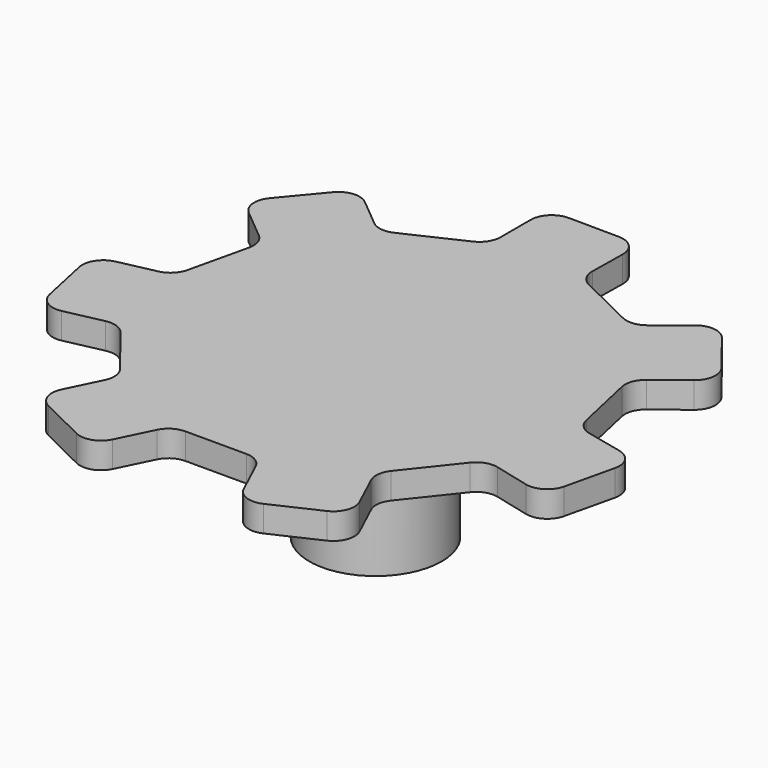
from build123d import *

# Parameters (mm, degrees)
F1_DEPTH  = 2.54
F2_SCALE  = 1.12
F3_R      = 1.27
F4_R      = 4.0005
F4_R_2    = 2.1462999284
F5_DEPTH  = 7.0104
F6_R      = 2.2083863112
F7_DEPTH  = 7.0104
F8_DEPTH  = 1.27
F9_R      = 5.1360331122
F10_DEPTH = 1.27


with BuildPart() as f1:
    # F0 (on Top) → F1 (new body)
    with BuildSketch(Plane.XY):
        Polygon((2.6097216178, 14.5627437159), (-2.4016266689, 14.6046923473), (-2.4016266689, 10.7069099322), (-6.7973635159, 8.6464090273), (-9.7507489845, 11.1018400639), (-12.9371215583, 7.269280193), (-9.9187448393, 4.759815731), (-10.987800546, 0.1461525389), (-14.7898914292, -0.6685812259), (-13.7329729143, -5.6008676039), (-9.9187448393, -4.7835330123), (-6.9650523365, -8.5103949532), (-8.662414737, -11.9730141014), (-4.136644538, -14.1915290003), (-2.4166579341, -10.6827564792), (2.3025460541, -10.6827564792), (3.9659612812, -14.2644541338), (8.5153820935, -12.1516080526), (6.8819414162, -8.6344521752), (9.8897544667, -4.8440932296), (13.6239528656, -5.7776425965), (14.7675592452, -0.8934023208), (10.9942825511, -0.0382388607), (9.9505092949, 4.6697063372), (13.008704409, 7.0334360935), (9.9016642198, 10.9836040065), (6.8838195875, 8.5752755404), (2.5481330231, 10.6975259259), align=None)
    extrude(amount=F1_DEPTH)


with BuildPart() as f1_1:
    # F2: moved
    add(f1.part.scale(F2_SCALE))

    # F3
    f3_edges = [f1_1.edges().sort_by_distance(p)[0] for p in [
        (-16.564678, -0.748811, 1.4224),
        (-12.306337, 0.163691, 1.4224),
        (-14.489576, 8.141594, 1.4224),
        (-10.920839, 12.434061, 1.4224),
        (-7.613047, 9.683978, 1.4224),
        (-2.689822, 11.991739, 1.4224),
        (-2.689822, 16.357255, 1.4224),
        (2.922888, 16.310273, 1.4224),
        (2.853909, 11.981229, 1.4224),
        (7.709878, 9.604309, 1.4224),
        (11.089864, 12.301636, 1.4224),
        (14.569749, 7.877448, 1.4224),
        (11.14457, 5.230071, 1.4224),
        (12.313596, -0.042828, 1.4224),
        (16.539666, -1.000611, 1.4224),
        (15.258827, -6.47096, 1.4224),
        (11.076525, -5.425384, 1.4224),
        (7.707774, -9.670586, 1.4224),
        (9.537228, -13.609801, 1.4224),
        (4.441877, -15.976189, 1.4224),
        (2.578852, -11.964687, 1.4224),
        (-2.706657, -11.964687, 1.4224),
        (-4.633042, -15.894512, 1.4224),
        (-9.701905, -13.409776, 1.4224),
        (-7.800859, -9.531642, 1.4224),
        (-11.108994, -5.357557, 1.4224),
        (-15.38093, -6.272972, 1.4224),
        (-11.108994, 5.330994, 1.4224),
    ]]
    fillet(f3_edges, radius=F3_R)

    # F4 (on face) → F5 (join)
    with BuildSketch(Plane.XY):
        Circle(F4_R)
        Circle(F4_R_2, mode=Mode.SUBTRACT)
        Circle(F4_R_2)
    extrude(amount=-F5_DEPTH)

    # F6 (on face) → F7 (cut)
    with BuildSketch(Plane(origin=(0, 0, -7.0104), x_dir=(1, 0, 0), z_dir=(0, 0, -1))):
        Circle(F6_R)
    extrude(amount=-F7_DEPTH, mode=Mode.SUBTRACT)

    # F8 (cut): a face of the model
    f8_faces = [f1_1.faces().sort_by_distance(p)[0] for p in [
        (5.0824398182, 10.382465325, 0),
    ]]
    extrude(f8_faces, amount=-F8_DEPTH, mode=Mode.SUBTRACT)

    # F9 (on face) → F10 (join)
    with BuildSketch(Plane.XY):
        Circle(F9_R)
    extrude(amount=F10_DEPTH)


solid = f1_1.part
